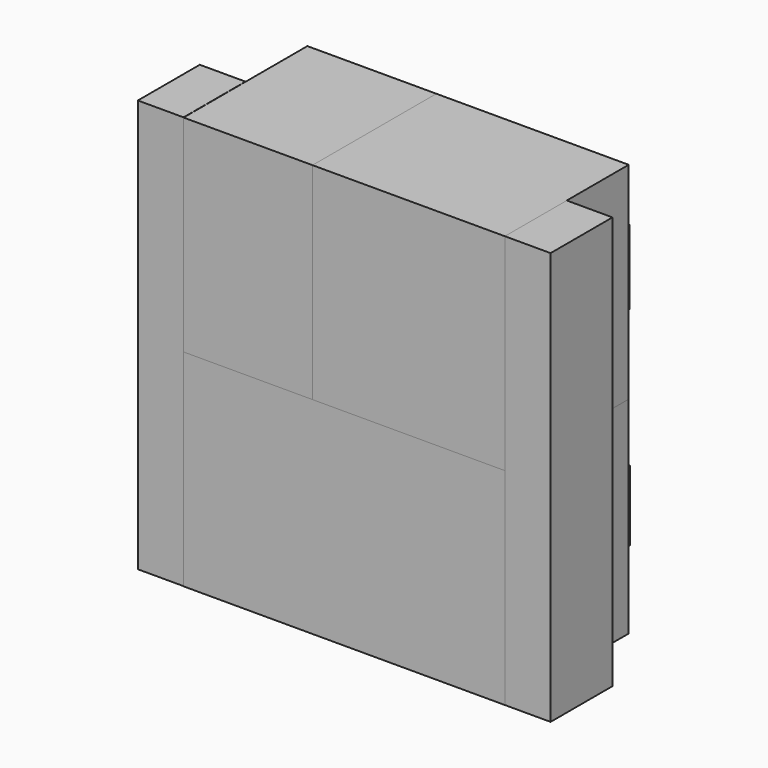
from build123d import *

# Parameters (mm, degrees)
F2_DEPTH       = 76.2
F3_DEPTH       = 76.2
F4_DEPTH       = 152.4
F0_W           = 189.39999966
F0_H           = 203.2
F5_DEPTH       = 152.4
F0_W_2         = 127
F6_DEPTH       = 152.4
F7_TEXT_SIZE   = 102.5681344358
F7_TEXT_SIZE_2 = 58.6692826049
F8_TEXT_SIZE   = 97.0784792092
F9_DEPTH       = 12.7


# Not quite as in the source:
# - Text() gives the source's letters only with a copy of the font that has no kerning and outlines rounded to 1/6400 em; it was checked with that copy


with BuildPart() as f2:
    # F1 (on face) → F2 (new body)
    with BuildSketch(Plane.XZ):
        Polygon((-180.6616566596, 203.2), (-180.6616566596, 203.369865787), (-225.6616566596, 203.369865787), (-225.6616566596, -203.030134213), (-180.6616566596, -203.030134213), (-180.6616566596, 0), align=None)
    extrude(amount=-F2_DEPTH)


with BuildPart() as f3:
    # F0 (on Front) → F3 (new body)
    with BuildSketch(Plane.XZ):
        Polygon((180.7383430004, 203.2), (135.7383430004, 203.2), (135.7383430004, 0), (135.7383430004, -203.2), (180.7383430004, -203.2), align=None)
    extrude(amount=-F3_DEPTH)


with BuildPart() as f4:
    # F0 (on Front) → F4 (new body)
    with BuildSketch(Plane.XZ):
        Polygon((135.7383430004, -203.2), (135.7383430004, 0), (-53.6616566596, 0), (-180.6616566596, 0), (-180.6616566596, -203.2), align=None)
    extrude(amount=-F4_DEPTH)


with BuildPart() as f5:
    # F0 (on Front) → F5 (new body)
    with BuildSketch(Plane.XZ):
        with Locations((41.0383431704, 101.6)):
            Rectangle(F0_W, F0_H)
    extrude(amount=-F5_DEPTH)


with BuildPart() as f6:
    # F0 (on Front) → F6 (new body)
    with BuildSketch(Plane.XZ):
        with Locations((-117.1616566596, 101.6)):
            Rectangle(F0_W_2, F0_H)
    extrude(amount=-F6_DEPTH)


with BuildPart() as f9:
    # F7 (on face) + F8 (on face) → F9 (new body)
    with BuildSketch(Plane(origin=(0, 152.4, 0), x_dir=(-1, 0, 0), z_dir=(0, 1, 0))):
        with Locations((-135.7383430004, 69.8382286891)):
            Text('Bin', F7_TEXT_SIZE, font='Open Sans', font_style=FontStyle.BOLD, text_align=(TextAlign.LEFT, TextAlign.BOTTOM))
        with Locations((53.6616566596, 111.8706939629)):
            Text('Arm', F7_TEXT_SIZE_2, font='Open Sans', font_style=FontStyle.BOLD, text_align=(TextAlign.LEFT, TextAlign.BOTTOM))
    with BuildSketch(Plane(origin=(0, 152.4, 0), x_dir=(-1, 0, 0), z_dir=(0, 1, 0))):
        with Locations((-135.7383430004, -134.765799422)):
            Text('Intake', F8_TEXT_SIZE, font='Open Sans', font_style=FontStyle.BOLD, text_align=(TextAlign.LEFT, TextAlign.BOTTOM))
    extrude(amount=F9_DEPTH)


solid = Compound([f2.part, f3.part, f4.part, f5.part, f6.part, f9.part])
